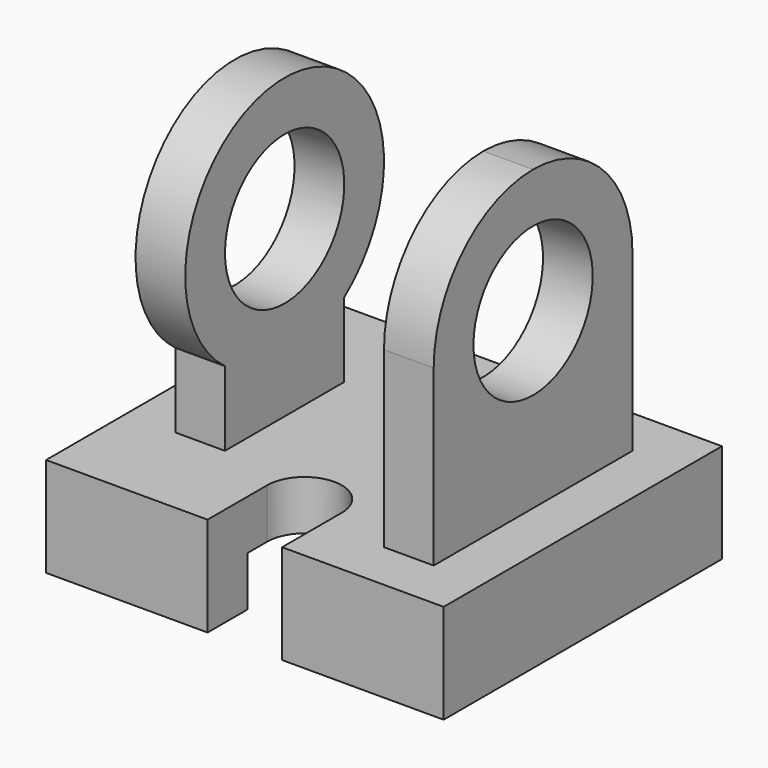
from build123d import *

# Parameters (mm, degrees)
F0_W      = 80
F0_H      = 70
F1_DEPTH  = 20
F2_W      = 60
F2_H      = 50
F3_DEPTH  = 10
F5_DEPTH  = 20.001
F6_W      = 10
F6_H      = 50
F7_DEPTH  = 60
F8_R      = 24.99999
F11_DEPTH = 10
F12_R     = 15
F13_DEPTH = 70.001


# Not quite as in the source:
# - a fillet or chamfer is up to 0.001 mm smaller than in the source, because OpenCascade refuses the exact size


with BuildPart() as f1:
    # F0 (on Top) → F1 (new body)
    with BuildSketch(Plane.XY):
        Rectangle(F0_W, F0_H)
    extrude(amount=F1_DEPTH)

    # F2 (on face) → F3 (cut)
    with BuildSketch(Plane(origin=(0, 0, 0), x_dir=(1, 0, 0), z_dir=(0, 0, -1))):
        Rectangle(F2_W, F2_H)
    extrude(amount=-F3_DEPTH, mode=Mode.SUBTRACT)

    # F4 (on face) → F5 (cut, through all)
    with BuildSketch(Plane.XY.offset(20)):
        with BuildLine():
            Line((7.5, -35), (7.5, -20))
            ThreePointArc((7.5, -20), (0, -12.5), (-7.5, -20))
            Line((-7.5, -20), (-7.5, -35))
            Line((-7.5, -35), (7.5, -35))
        make_face()
    extrude(amount=-F5_DEPTH, mode=Mode.SUBTRACT)

    # F6 (on face) → F7 (join)
    with BuildSketch(Plane.XY.offset(20)):
        with Locations((25, 0)):
            Rectangle(F6_W, F6_H)
    extrude(amount=F7_DEPTH)

    # F8 (radius 25 in the source; OpenCascade refuses exactly that, so slightly less here)
    f8_edges = [f1.edges().sort_by_distance(p)[0] for p in [
        (25, -25, 80),
        (25, 25, 80),
    ]]
    fillet(f8_edges, radius=F8_R)

    # F10 (on offset) → F11 (join)
    with BuildSketch(Plane(origin=(-30, 0, 0), x_dir=(0, -1, 0), z_dir=(-1, 0, 0))):
        with BuildLine():
            Line((15, 20), (15, 35))
            ThreePointArc((15, 35), (0, 80), (-15, 35))
            Line((-15, 35), (-15, 20))
            Line((-15, 20), (15, 20))
        make_face()
    extrude(amount=-F11_DEPTH)

    # F12 (on face) → F13 (cut, through all)
    with BuildSketch(Plane(origin=(-30, 0, 0), x_dir=(0, -1, 0), z_dir=(-1, 0, 0))):
        with Locations((0, 55)):
            Circle(F12_R)
    extrude(amount=-F13_DEPTH, mode=Mode.SUBTRACT)


solid = f1.part
